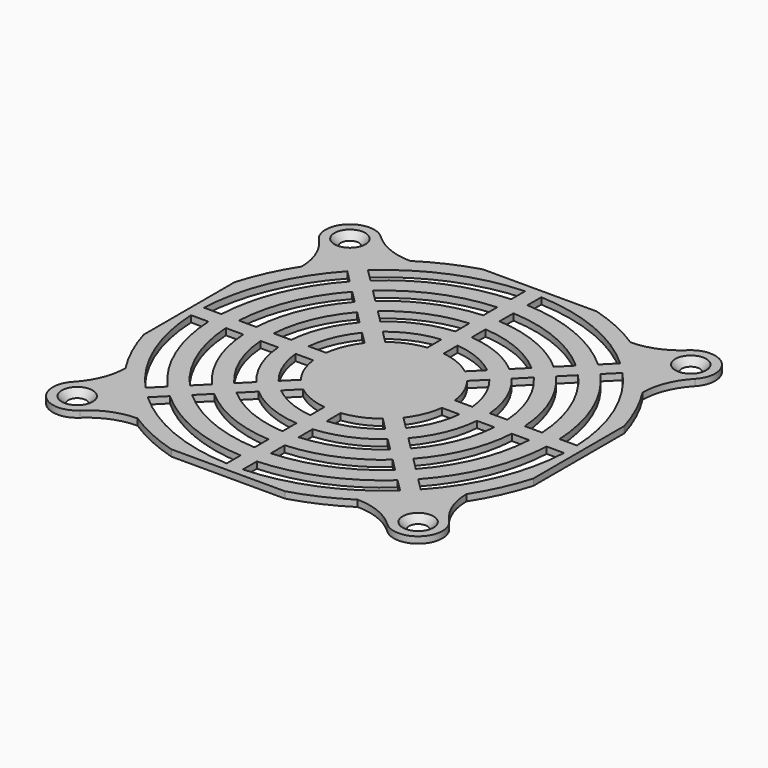
from build123d import *

# Parameters (mm, degrees)
F0_R     = 2.75
F1_DEPTH = 2
F2_SIZE  = 1.99999
F4_DEPTH = 2
F6_DEPTH = 2


# Not quite as in the source:
# - a fillet or chamfer is up to 0.001 mm smaller than in the source, because OpenCascade refuses the exact size


with BuildPart() as f1:
    # F0 (on Top) → F1 (new body)
    with BuildSketch(Plane.XY):
        with BuildLine():
            ThreePointArc((54.3529411765, 25.4117647059), (52.7572589097, 36.9222842596), (57.9310344828, 47.3275862069))
            ThreePointArc((57.9310344828, 47.3275862069), (57.8033008589, 57.8033008589), (47.3275862069, 57.9310344828))
            ThreePointArc((47.3275862069, 57.9310344828), (36.9222842596, 52.7572589097), (25.4117647059, 54.3529411765))
            ThreePointArc((25.4117647059, 54.3529411765), (0, 60), (-25.4117647059, 54.3529411765))
            ThreePointArc((-25.4117647059, 54.3529411765), (-36.9222842596, 52.7572589097), (-47.3275862069, 57.9310344828))
            ThreePointArc((-47.3275862069, 57.9310344828), (-57.8033008589, 57.8033008589), (-57.9310344828, 47.3275862069))
            ThreePointArc((-57.9310344828, 47.3275862069), (-52.7572589097, 36.9222842596), (-54.3529411765, 25.4117647059))
            ThreePointArc((-54.3529411765, 25.4117647059), (-60, 0), (-54.3529411765, -25.4117647059))
            ThreePointArc((-54.3529411765, -25.4117647059), (-52.7572589097, -36.9222842596), (-57.9310344828, -47.3275862069))
            ThreePointArc((-57.9310344828, -47.3275862069), (-57.8033008589, -57.8033008589), (-47.3275862069, -57.9310344828))
            ThreePointArc((-47.3275862069, -57.9310344828), (-36.9222842596, -52.7572589097), (-25.4117647059, -54.3529411765))
            ThreePointArc((-25.4117647059, -54.3529411765), (0, -60), (25.4117647059, -54.3529411765))
            ThreePointArc((25.4117647059, -54.3529411765), (36.9222842596, -52.7572589097), (47.3275862069, -57.9310344828))
            ThreePointArc((47.3275862069, -57.9310344828), (57.8033008589, -57.8033008589), (57.9310344828, -47.3275862069))
            ThreePointArc((57.9310344828, -47.3275862069), (52.7572589097, -36.9222842596), (54.3529411765, -25.4117647059))
            ThreePointArc((54.3529411765, -25.4117647059), (60, 0), (54.3529411765, 25.4117647059))
        make_face()
        with Locations((-52.5, -52.5)):
            Circle(F0_R, mode=Mode.SUBTRACT)
        with BuildLine():
            ThreePointArc((-2.5, -57.4456264654), (-40.6586399182, -40.6586399182), (-57.4456264654, -2.5))
            Line((-57.4456264654, -2.5), (-52.0828911546, -2.5))
            ThreePointArc((-52.0828911546, -2.5), (-36.8705678762, -36.8705678762), (-2.5, -52.0828911546))
            Line((-2.5, -52.0828911546), (-2.5, -57.4456264654))
        make_face(mode=Mode.SUBTRACT)
        with BuildLine():
            ThreePointArc((-2.5, -46.7188726451), (-33.0824958341, -33.0824958341), (-46.7188726451, -2.5))
            Line((-46.7188726451, -2.5), (-41.3530715983, -2.5))
            ThreePointArc((-41.3530715983, -2.5), (-29.294423792, -29.294423792), (-2.5, -41.3530715983))
            Line((-2.5, -41.3530715983), (-2.5, -46.7188726451))
        make_face(mode=Mode.SUBTRACT)
        with BuildLine():
            ThreePointArc((-2.5, -35.9846906223), (-25.5063517499, -25.5063517499), (-35.9846906223, -2.5))
            Line((-35.9846906223, -2.5), (-30.6123724487, -2.5))
            ThreePointArc((-30.6123724487, -2.5), (-21.7182797079, -21.7182797079), (-2.5, -30.6123724487))
            Line((-2.5, -30.6123724487), (-2.5, -35.9846906223))
        make_face(mode=Mode.SUBTRACT)
        with BuildLine():
            ThreePointArc((-2.5, -25.2336024752), (-17.9302076658, -17.9302076658), (-25.2336024752, -2.5))
            Line((-25.2336024752, -2.5), (-19.843134833, -2.5))
            ThreePointArc((-19.843134833, -2.5), (-14.1421356237, -14.1421356237), (-2.5, -19.843134833))
            Line((-2.5, -19.843134833), (-2.5, -25.2336024752))
        make_face(mode=Mode.SUBTRACT)
        with Locations((52.5, -52.5)):
            Circle(F0_R, mode=Mode.SUBTRACT)
        with BuildLine():
            Line((52.0828911546, -2.5), (57.4456264654, -2.5))
            ThreePointArc((57.4456264654, -2.5), (40.6586399182, -40.6586399182), (2.5, -57.4456264654))
            Line((2.5, -57.4456264654), (2.5, -52.0828911546))
            ThreePointArc((2.5, -52.0828911546), (36.8705678762, -36.8705678762), (52.0828911546, -2.5))
        make_face(mode=Mode.SUBTRACT)
        with BuildLine():
            Line((41.3530715983, -2.5), (46.7188726451, -2.5))
            ThreePointArc((46.7188726451, -2.5), (33.0824958341, -33.0824958341), (2.5, -46.7188726451))
            Line((2.5, -46.7188726451), (2.5, -41.3530715983))
            ThreePointArc((2.5, -41.3530715983), (29.294423792, -29.294423792), (41.3530715983, -2.5))
        make_face(mode=Mode.SUBTRACT)
        with BuildLine():
            Line((30.6123724487, -2.5), (35.9846906223, -2.5))
            ThreePointArc((35.9846906223, -2.5), (25.5063517499, -25.5063517499), (2.5, -35.9846906223))
            Line((2.5, -35.9846906223), (2.5, -30.6123724487))
            ThreePointArc((2.5, -30.6123724487), (21.7182797079, -21.7182797079), (30.6123724487, -2.5))
        make_face(mode=Mode.SUBTRACT)
        with BuildLine():
            Line((19.843134833, -2.5), (25.2336024752, -2.5))
            ThreePointArc((25.2336024752, -2.5), (17.9302076658, -17.9302076658), (2.5, -25.2336024752))
            Line((2.5, -25.2336024752), (2.5, -19.843134833))
            ThreePointArc((2.5, -19.843134833), (14.1421356237, -14.1421356237), (19.843134833, -2.5))
        make_face(mode=Mode.SUBTRACT)
        with BuildLine():
            ThreePointArc((-2.5, 19.843134833), (-14.1421356237, 14.1421356237), (-19.843134833, 2.5))
            Line((-19.843134833, 2.5), (-25.2336024752, 2.5))
            ThreePointArc((-25.2336024752, 2.5), (-17.9302076658, 17.9302076658), (-2.5, 25.2336024752))
            Line((-2.5, 25.2336024752), (-2.5, 19.843134833))
        make_face(mode=Mode.SUBTRACT)
        with BuildLine():
            Line((-30.6123724487, 2.5), (-35.9846906223, 2.5))
            ThreePointArc((-35.9846906223, 2.5), (-25.5063517499, 25.5063517499), (-2.5, 35.9846906223))
            Line((-2.5, 35.9846906223), (-2.5, 30.6123724487))
            ThreePointArc((-2.5, 30.6123724487), (-21.7182797079, 21.7182797079), (-30.6123724487, 2.5))
        make_face(mode=Mode.SUBTRACT)
        with BuildLine():
            Line((-41.3530715983, 2.5), (-46.7188726451, 2.5))
            ThreePointArc((-46.7188726451, 2.5), (-33.0824958341, 33.0824958341), (-2.5, 46.7188726451))
            Line((-2.5, 46.7188726451), (-2.5, 41.3530715983))
            ThreePointArc((-2.5, 41.3530715983), (-29.294423792, 29.294423792), (-41.3530715983, 2.5))
        make_face(mode=Mode.SUBTRACT)
        with BuildLine():
            Line((-52.0828911546, 2.5), (-57.4456264654, 2.5))
            ThreePointArc((-57.4456264654, 2.5), (-40.6586399182, 40.6586399182), (-2.5, 57.4456264654))
            Line((-2.5, 57.4456264654), (-2.5, 52.0828911546))
            ThreePointArc((-2.5, 52.0828911546), (-36.8705678762, 36.8705678762), (-52.0828911546, 2.5))
        make_face(mode=Mode.SUBTRACT)
        with Locations((-52.5, 52.5)):
            Circle(F0_R, mode=Mode.SUBTRACT)
        with BuildLine():
            Line((25.2336024752, 2.5), (19.843134833, 2.5))
            ThreePointArc((19.843134833, 2.5), (14.1421356237, 14.1421356237), (2.5, 19.843134833))
            Line((2.5, 19.843134833), (2.5, 25.2336024752))
            ThreePointArc((2.5, 25.2336024752), (17.9302076658, 17.9302076658), (25.2336024752, 2.5))
        make_face(mode=Mode.SUBTRACT)
        with BuildLine():
            Line((35.9846906223, 2.5), (30.6123724487, 2.5))
            ThreePointArc((30.6123724487, 2.5), (21.7182797079, 21.7182797079), (2.5, 30.6123724487))
            Line((2.5, 30.6123724487), (2.5, 35.9846906223))
            ThreePointArc((2.5, 35.9846906223), (25.5063517499, 25.5063517499), (35.9846906223, 2.5))
        make_face(mode=Mode.SUBTRACT)
        with BuildLine():
            Line((46.7188726451, 2.5), (41.3530715983, 2.5))
            ThreePointArc((41.3530715983, 2.5), (29.294423792, 29.294423792), (2.5, 41.3530715983))
            Line((2.5, 41.3530715983), (2.5, 46.7188726451))
            ThreePointArc((2.5, 46.7188726451), (33.0824958341, 33.0824958341), (46.7188726451, 2.5))
        make_face(mode=Mode.SUBTRACT)
        with BuildLine():
            Line((57.4456264654, 2.5), (52.0828911546, 2.5))
            ThreePointArc((52.0828911546, 2.5), (36.8705678762, 36.8705678762), (2.5, 52.0828911546))
            Line((2.5, 52.0828911546), (2.5, 57.4456264654))
            ThreePointArc((2.5, 57.4456264654), (40.6586399182, 40.6586399182), (57.4456264654, 2.5))
        make_face(mode=Mode.SUBTRACT)
        with Locations((52.5, 52.5)):
            Circle(F0_R, mode=Mode.SUBTRACT)
    extrude(amount=F1_DEPTH)

    # F2 (size 2 in the source; OpenCascade refuses exactly that, so slightly less here)
    f2_edges = [f1.edges().sort_by_distance(p)[0] for p in [
        (-55.25, -52.5, 2),
        (-55.25, 52.5, 2),
        (49.75, 52.5, 2),
        (49.75, -52.5, 2),
    ]]
    chamfer(f2_edges, length=F2_SIZE)

    # F3 (on face) → F4 (join)
    with BuildSketch(Plane.XY.offset(2)):
        Polygon((-44.1245098269, 47.6600437328), (-47.6600437328, 44.1245098269), (-3.5355339059, 0), (0, 3.5355339059), align=None)
        Polygon((0, 3.5355339059), (-3.5355339059, 0), (0, -3.5355339059), (3.5355339059, 0), align=None)
        Polygon((0, -3.5355339059), (-3.5355339059, 0), (-47.6600437328, -44.1245098269), (-44.1245098269, -47.6600437328), align=None)
        Polygon((3.5355339059, 0), (0, -3.5355339059), (44.1245098269, -47.6600437328), (47.6600437328, -44.1245098269), align=None)
        Polygon((44.1245098269, 47.6600437328), (0, 3.5355339059), (3.5355339059, 0), (47.6600437328, 44.1245098269), align=None)
    extrude(amount=-F4_DEPTH)

    # F5 (on face) → F6 (join)
    with BuildSketch(Plane.XY.offset(2)):
        with BuildLine():
            ThreePointArc((-33.9106353307, -52.5006553432), (-25.9773632004, -56.8456383652), (-17.5, -60))
            Line((-17.5, -60), (-1.711e-07, -60))
            ThreePointArc((-1.711e-07, -60), (-13.0158275526, -58.5712235925), (-25.4117647059, -54.3529411765))
            ThreePointArc((-25.4117647059, -54.3529411765), (-29.5576228709, -52.9515536948), (-33.9106353307, -52.5006553432))
        make_face()
        with BuildLine():
            ThreePointArc((17.5, -60), (25.9773632004, -56.8456383652), (33.9106353307, -52.5006553432))
            ThreePointArc((33.9106353307, -52.5006553432), (29.5576228709, -52.9515536948), (25.4117647059, -54.3529411765))
            ThreePointArc((25.4117647059, -54.3529411765), (13.0158273856, -58.5712236296), (-1.711e-07, -60))
            Line((-1.711e-07, -60), (17.5, -60))
        make_face()
        with BuildLine():
            ThreePointArc((-60, -17.5), (-56.8456383652, -25.9773632004), (-52.5006553432, -33.9106353307))
            ThreePointArc((-52.5006553432, -33.9106353307), (-52.9515536948, -29.5576228709), (-54.3529411765, -25.4117647059))
            ThreePointArc((-54.3529411765, -25.4117647059), (-58.5712236368, -13.0158273533), (-60, 2.373e-07))
            Line((-60, 2.373e-07), (-60, -17.5))
        make_face()
        with BuildLine():
            ThreePointArc((-54.3529411765, 25.4117647059), (-52.9515536948, 29.5576228709), (-52.5006553432, 33.9106353307))
            ThreePointArc((-52.5006553432, 33.9106353307), (-56.8456383652, 25.9773632004), (-60, 17.5))
            Line((-60, 17.5), (-60, 2.373e-07))
            ThreePointArc((-60, 2.373e-07), (-58.5712235853, 13.015827585), (-54.3529411765, 25.4117647059))
        make_face()
        with BuildLine():
            Line((8.08e-08, 60), (-17.5, 60))
            ThreePointArc((-17.5, 60), (-25.9773632004, 56.8456383652), (-33.9106353307, 52.5006553432))
            ThreePointArc((-33.9106353307, 52.5006553432), (-29.5576228709, 52.9515536948), (-25.4117647059, 54.3529411765))
            ThreePointArc((-25.4117647059, 54.3529411765), (-13.0158274297, 58.5712236198), (8.08e-08, 60))
        make_face()
        with BuildLine():
            ThreePointArc((25.4117647059, 54.3529411765), (29.5576228709, 52.9515536948), (33.9106353307, 52.5006553432))
            ThreePointArc((33.9106353307, 52.5006553432), (25.9773632004, 56.8456383652), (17.5, 60))
            Line((17.5, 60), (8.08e-08, 60))
            ThreePointArc((8.08e-08, 60), (13.0158275086, 58.5712236023), (25.4117647059, 54.3529411765))
        make_face()
        with BuildLine():
            Line((60, 0), (60, 17.5))
            ThreePointArc((60, 17.5), (56.8456383652, 25.9773632004), (52.5006553432, 33.9106353307))
            ThreePointArc((52.5006553432, 33.9106353307), (52.9515536948, 29.5576228709), (54.3529411765, 25.4117647059))
            ThreePointArc((54.3529411765, 25.4117647059), (58.571223611, 13.0158274691), (60, 0))
        make_face()
        with BuildLine():
            ThreePointArc((52.5006553432, -33.9106353307), (56.8456383652, -25.9773632004), (60, -17.5))
            Line((60, -17.5), (60, 0))
            ThreePointArc((60, 0), (58.571223611, -13.0158274691), (54.3529411765, -25.4117647059))
            ThreePointArc((54.3529411765, -25.4117647059), (52.9515536948, -29.5576228709), (52.5006553432, -33.9106353307))
        make_face()
    extrude(amount=-F6_DEPTH)


solid = f1.part
